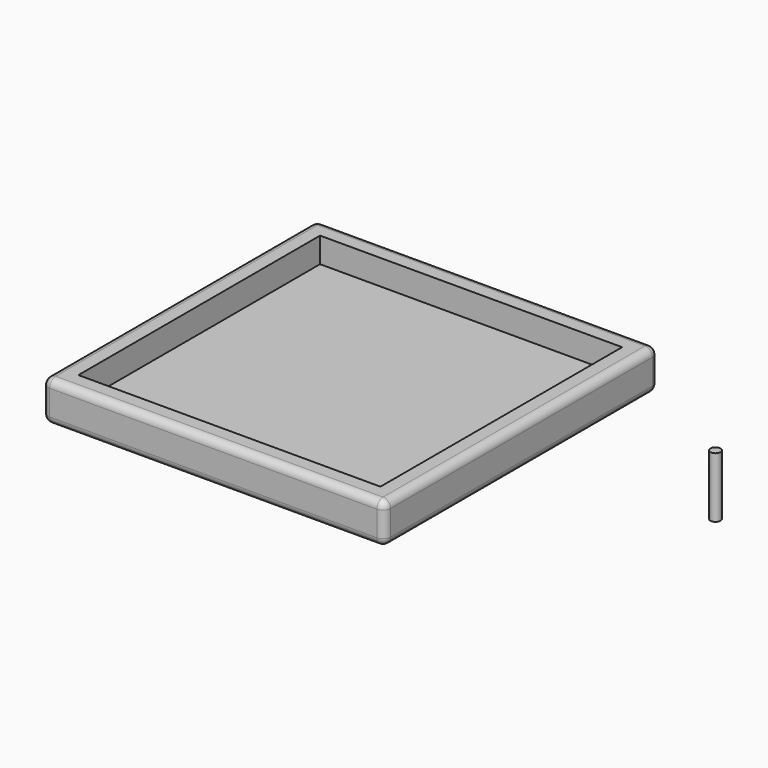
from build123d import *

# Parameters (mm, degrees)
F0_W      = 340
F0_H      = 340
F0_W_2    = 300
F0_H_2    = 300
F1_DEPTH  = 40
F2_DEPTH  = 5
F3_W      = 15
F3_H      = 20
F4_DEPTH  = 80
F5_R      = 9.99999
F6_R      = 7.5
F7_R      = 5
F8_DEPTH  = 45
F0_R      = 5
F10_DEPTH = 60
F3_W_2    = 127.5
F3_H_2    = 140
F11_DEPTH = 60.001
F12_W     = 127.5
F12_H     = 140
F13_DEPTH = 10


# Not quite as in the source:
# - a fillet or chamfer is up to 0.001 mm smaller than in the source, because OpenCascade refuses the exact size


with BuildPart() as f1:
    # F0 (on Top) → F1 (new body)
    with BuildSketch(Plane.XY):
        Rectangle(F0_W, F0_H)
        Rectangle(F0_W_2, F0_H_2, mode=Mode.SUBTRACT)
    extrude(amount=F1_DEPTH)

    # F0 (on Top) → F2 (join)
    with BuildSketch(Plane.XY):
        Rectangle(F0_W_2, F0_H_2)
    extrude(amount=F2_DEPTH)

    # F3 (on face) → F4 (join)
    with BuildSketch(Plane.XY):
        with Locations((15, 0)):
            Rectangle(F3_W, F3_H)
        with Locations((-15, 0)):
            Rectangle(F3_W, F3_H)
    extrude(amount=-F4_DEPTH)

    # F5 (radius 10 in the source; OpenCascade refuses exactly that, so slightly less here)
    f5_edges = [f1.edges().sort_by_distance(p)[0] for p in [
        (-15, -10, -80),
        (-15, 10, -80),
        (15, -10, -80),
        (15, 10, -80),
    ]]
    fillet(f5_edges, radius=F5_R)

    # F6
    f6_edges = [f1.edges().sort_by_distance(p)[0] for p in [
        (-170, -170, 20),
        (170, -170, 20),
        (-170, 170, 20),
        (0, 170, 0),
        (170, 0, 0),
        (170, 170, 20),
        (170, 0, 40),
        (0, -170, 40),
        (0, -170, 0),
        (-170, 0, 40),
        (-170, 0, 0),
        (0, 170, 40),
    ]]
    fillet(f6_edges, radius=F6_R)


with BuildPart() as f8:
    # F7 (on face) → F8 (new body)
    with BuildSketch(Plane(origin=(-22.5, 0, 0), x_dir=(0, -1, 0), z_dir=(-1, 0, 0))):
        with Locations((0, -70)):
            Circle(F7_R)
    extrude(amount=-F8_DEPTH)


with BuildPart() as f1_1:
    add(f1.part)

    # F9: cut F8
    add(f8.part, mode=Mode.SUBTRACT)

    # F3 (on face) → F11 (cut, through all)
    with BuildSketch(Plane.XY):
        with Locations((-86.25, 80)):
            Rectangle(F3_W_2, F3_H_2)
        with Locations((86.25, 80)):
            Rectangle(F3_W_2, F3_H_2)
        with Locations((86.25, -80)):
            Rectangle(F3_W_2, F3_H_2)
        with Locations((-86.25, -80)):
            Rectangle(F3_W_2, F3_H_2)
    extrude(amount=F11_DEPTH, mode=Mode.SUBTRACT)


with BuildPart() as f10:
    # F0 (on Top) → F10 (new body)
    with BuildSketch(Plane.XY):
        with Locations((338.7121260166, 30.0132371485)):
            Circle(F0_R)
    extrude(amount=F10_DEPTH)


with BuildPart() as f13:
    # F12 (on face) → F13 (new body)
    with BuildSketch(Plane.XY.offset(5)):
        with Locations((86.25, 80)):
            Rectangle(F12_W, F12_H)
        Polygon((22.5, 10), (22.5, 150), (-22.5, 150), (-22.5, 10), (-150, 10), (-150, -10), (-22.5, -10), (-22.5, -150), (22.5, -150), (22.5, -10), (150, -10), (150, 10), align=None)
        with Locations((-86.25, 80)):
            Rectangle(F12_W, F12_H)
        with Locations((86.25, -80)):
            Rectangle(F12_W, F12_H)
        with Locations((-86.25, -80)):
            Rectangle(F12_W, F12_H)
    extrude(amount=F13_DEPTH)


solid = Compound([f1_1.part, f10.part, f13.part])
